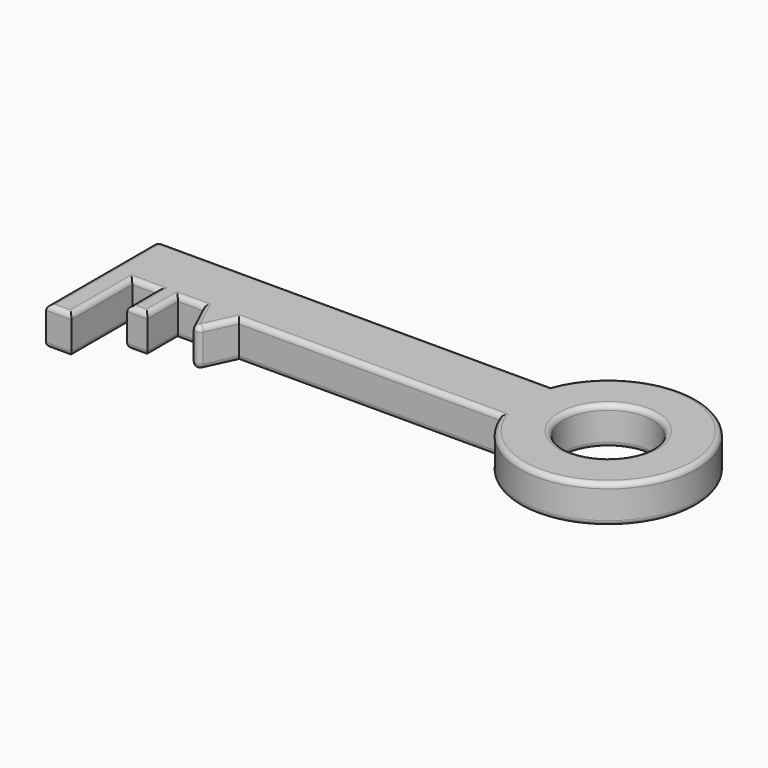
from build123d import *

# Parameters (mm, degrees)
F0_W     = 10
F0_H     = 30
F0_W_2   = 8
F0_H_2   = 15
F1_DEPTH = 15
F2_R     = 2


# Not quite as in the source:
# - a feature of the source that left no trace in its solid (it failed there, or was rolled back) is left out


with BuildPart() as f1:
    # F0 (on Top) → F1 (new body)
    with BuildSketch(Plane.XY):
        Polygon((-60.840103223, 15), (-53.840103223, 30), (-67.840103223, 30), align=None)
        with Locations((-100.840103223, 15)):
            Rectangle(F0_W, F0_H)
        with Locations((-81.840103223, 22.5)):
            Rectangle(F0_W_2, F0_H_2)
        with BuildLine():
            ThreePointArc((49.159896777, 30), (116.8516388535, 42.5), (49.159896777, 55))
            Line((49.159896777, 55), (49.159896777, 42.5))
            Line((49.159896777, 42.5), (49.159896777, 30))
        make_face()
        with BuildLine():
            ThreePointArc((99.3516388535, 42.5), (81.8516388535, 25), (64.3516388535, 42.5))
            ThreePointArc((64.3516388535, 42.5), (81.8516388535, 60), (99.3516388535, 42.5))
        make_face(mode=Mode.SUBTRACT)
        Polygon((33.3130955696, 42.5), (-105.840103223, 42.5), (-105.840103223, 30), (-95.840103223, 30), (-85.840103223, 30), (-77.840103223, 30), (-67.840103223, 30), (-53.840103223, 30), (49.159896777, 30), (49.159896777, 42.5), align=None)
        Polygon((49.159896777, 55), (-105.840103223, 55), (-105.840103223, 42.5), (33.3130955696, 42.5), (49.159896777, 42.5), align=None)
    extrude(amount=F1_DEPTH)

    # F2
    f2_edges = [f1.edges().sort_by_distance(p)[0] for p in [
        (-28.340103, 55, 15),
        (-100.840103, 0, 15),
        (-105.840103, 27.5, 15),
        (-90.840103, 30, 15),
        (-95.840103, 15, 15),
        (-85.840103, 22.5, 15),
        (-81.840103, 15, 15),
        (-77.840103, 22.5, 15),
        (-72.840103, 30, 15),
        (-64.340103, 22.5, 15),
        (-2.340103, 30, 15),
        (116.851639, 42.5, 15),
        (99.351639, 42.5, 15),
        (-57.340103, 22.5, 0),
        (-105.840103, 27.5, 0),
        (116.851639, 42.5, 0),
        (-2.340103, 30, 0),
        (-81.840103, 15, 0),
        (-77.840103, 22.5, 0),
        (-95.840103, 15, 0),
        (-100.840103, 0, 0),
        (99.351639, 42.5, 0),
        (-28.340103, 55, 0),
        (-105.840103, 55, 7.5),
        (-64.340103, 22.5, 0),
        (-60.840103, 15, 7.5),
        (-57.340103, 22.5, 15),
        (-90.840103, 30, 0),
        (-85.840103, 22.5, 0),
        (-72.840103, 30, 0),
    ]]
    fillet(f2_edges, radius=F2_R)


solid = f1.part
